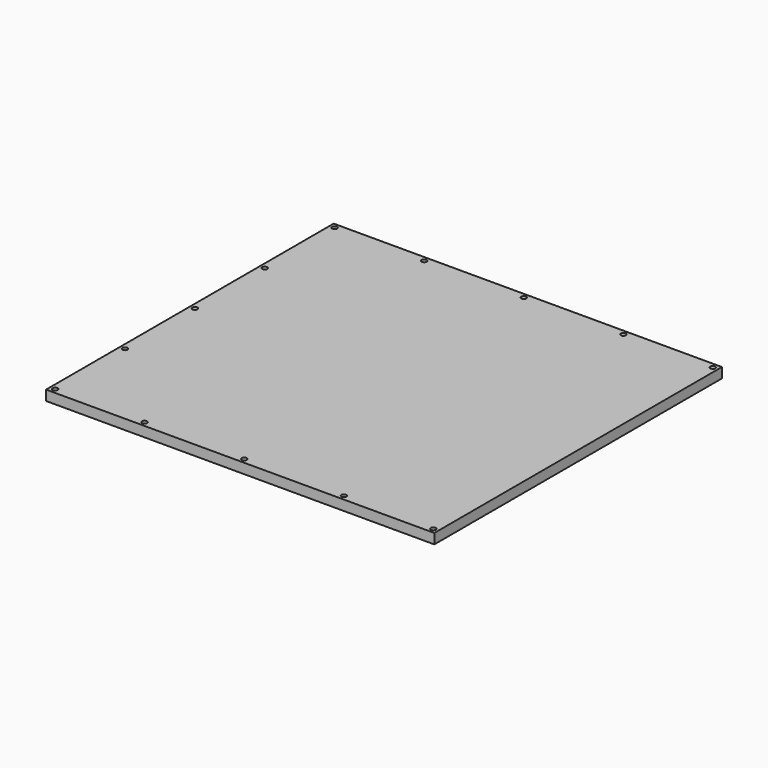
from build123d import *

# Parameters (mm, degrees)
F0_W            = 270
F0_H            = 250
F4_REACH        = 517.9673898595
F5_W            = 263
F5_H            = 236
F6_DEPTH        = 36
F8_DEPTH        = 250.001
F10_D           = 3.5
F10_DEPTH       = 12
F10_TIP         = 1.0515060833
F13_W           = 270
F13_H           = 250
F14_DEPTH       = 7
F15_D           = 3.5
F15_CSINK_D     = 5
F15_CSINK_ANGLE = 90


with BuildPart() as f4:
    f4_end = Plane(origin=(25.6515107494, 0, -145.4769465589), x_dir=(0.984807753, 0, 0.1736481777), z_dir=(-0.1736481777, 0, 0.984807753))
    # F0 (on Top) → F4 (new body, up to a plane its end follows)
    with BuildSketch(Plane.XY):
        with Locations((135, 125)):
            Rectangle(F0_W, F0_H)
    f4_long = extrude(amount=-F4_REACH, mode=Mode.PRIVATE)
    add(split(f4_long, bisect_by=f4_end, keep=Keep.TOP, mode=Mode.PRIVATE))

    # F5 (on face) → F6 (cut)
    with BuildSketch(Plane.XY):
        with Locations((138.5, 125)):
            Rectangle(F5_W, F5_H)
    extrude(amount=-F6_DEPTH, mode=Mode.SUBTRACT)

    # F7 (on face) → F8 (cut, through all)
    with BuildSketch(Plane.XZ):
        with BuildLine():
            Line((270, -42.8751187269), (216.5270364467, -52.3038449398))
            ThreePointArc((216.5270364467, -52.3038449398), (200.3038449398, -75.4729635533), (223.4729635533, -91.6961550602))
            Line((223.4729635533, -91.6961550602), (270, -83.4921832023))
            Line((270, -83.4921832023), (270, -42.8751187269))
        make_face()
    extrude(amount=-F8_DEPTH, mode=Mode.SUBTRACT)

    # F10
    with Locations(Plane.XY):
        with Locations((3.5, 64.25), (3.5, 125), (3.5, 185.75), (3.5, 246.5), (3.5, 3.5), (65.75, 3.5), (135, 3.5), (204.25, 3.5), (266.5, 3.5), (266.500000929, 246.5237677097), (204.25, 246.5237677097), (135, 246.5237677097), (65.75, 246.5)):
            Hole(F10_D / 2, depth=F10_DEPTH)
            with Locations((0, 0, -(F10_DEPTH + F10_TIP / 2))):  # 118° drill point
                Cone(0, F10_D / 2, F10_TIP, mode=Mode.SUBTRACT)


with BuildPart() as f14:
    # F13 (on face) → F14 (new body)
    with BuildSketch(Plane.XY):
        with Locations((135, 125)):
            Rectangle(F13_W, F13_H)
    extrude(amount=F14_DEPTH)

    # F15 (through all)
    with Locations(Plane(origin=(0, 0, 0), x_dir=(1, 0, 0), z_dir=(0, 0, -1))):
        with Locations((3.5, -246.5), (65.75, -246.5), (135, -246.5237677097), (204.25, -246.5237677097), (266.500000929, -246.5237677097), (3.5, -185.75), (3.5, -125), (3.5, -64.25), (3.5, -3.5), (65.75, -3.5), (135, -3.5), (204.25, -3.5), (266.5, -3.5)):
            CounterSinkHole(F15_D / 2, F15_CSINK_D / 2, counter_sink_angle=F15_CSINK_ANGLE)


solid = f14.part
